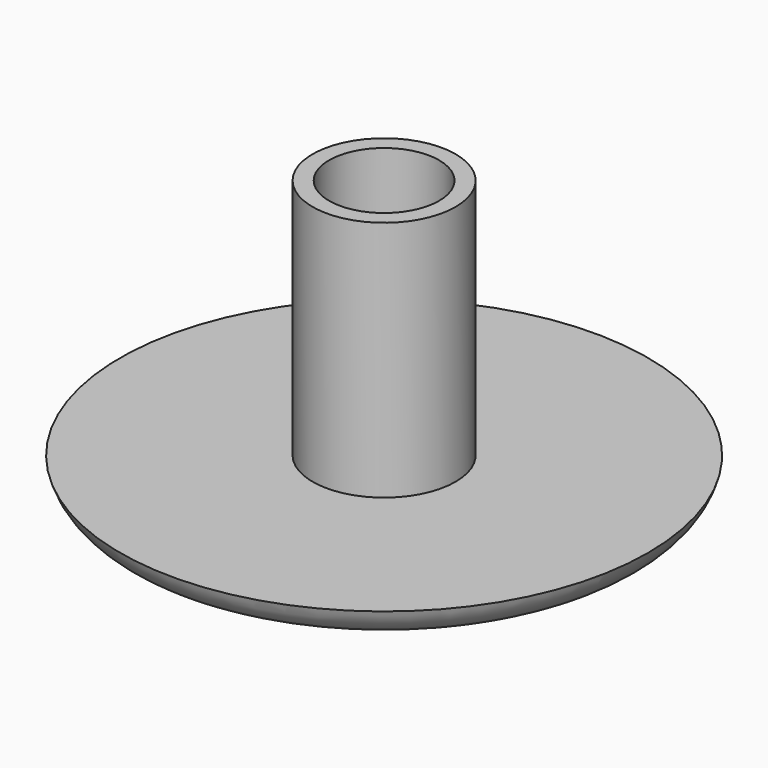
from build123d import *

# Parameters (mm, degrees)
F0_R     = 24
F0_R_2   = 6.5
F1_DEPTH = 3
F0_R_3   = 5
F2_DEPTH = 25
F3_R     = 7


# Not quite as in the source:
# - a fillet or chamfer that OpenCascade refuses, or shapes differently, is made with other operations: its cross-section is extruded or revolved along the edge and cut away or added


with BuildPart() as f1:
    # F0 (on Top) → F1 (new body)
    with BuildSketch(Plane.XY):
        Circle(F0_R)
        Circle(F0_R_2, mode=Mode.SUBTRACT)
    extrude(amount=F1_DEPTH)

    # F0 (on Top) → F2 (join)
    with BuildSketch(Plane.XY):
        Circle(F0_R_2)
        Circle(F0_R_3, mode=Mode.SUBTRACT)
    extrude(amount=F2_DEPTH)

    # F3
    f3_edges = [f1.edges().sort_by_distance(p)[0] for p in [
        (-5, 0, 0),
    ]]
    fillet(f3_edges, radius=F3_R)

    # F4: fillet of radius 4.104163056 on 1 edges, made by hand

    # F4_s1 → F4_t2 (revolve, cut)
    with BuildSketch(Plane.XZ):
        with BuildLine():
            ThreePointArc((20.0471556651, 0), (22.5283337288, 0.8349261716), (24, 3))
            Line((24, 3), (24, 0))
            Line((24, 0), (20.0471556651, 0))
        make_face()
    revolve(axis=Axis((0, 0, 0), (0, 0, 1)), mode=Mode.SUBTRACT)


solid = f1.part
